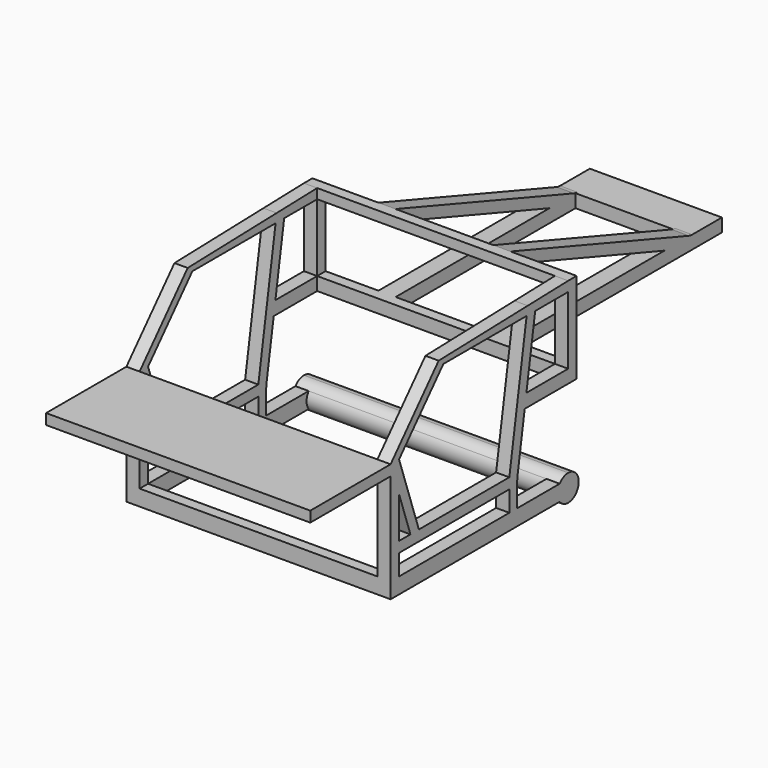
from build123d import *

# Parameters (mm, degrees)
F0_W     = 4
F0_H     = 6
F0_W_2   = 5.376602
F0_H_2   = 4
F0_W_3   = 3.587166
F0_H_3   = 7.83267
F0_H_4   = 5
F0_W_4   = 38
F1_DEPTH = 50
F2_DEPTH = 45
F3_DEPTH = 45
F4_DEPTH = 45
F5_DEPTH = 25
F6_DEPTH = 18.5
F7_W     = 14.907549
F7_H     = 5
F8_DEPTH = 37
F9_R     = 5


with BuildPart() as f1:
    # F0 (on Right) → F1 (new body, symmetric)
    with BuildSketch(Plane.YZ):
        Polygon((-49, -26), (-45, -26), (-45, -18.16733), (-45, -14.16733), (-45, 1.410587), (-49, 13), (-49, 9), align=None)
        with Locations((-47, -29)):
            Rectangle(F0_W, F0_H)
        Polygon((-26.269564, 38.284922), (-49, 13), (-45, 13), (-24.038542, 36.279295), align=None)
        Polygon((-24.038542, 36.279295), (15.345107, 36.279295), (15.861475, 39.464268), (-26.269564, 38.284922), align=None)
        Polygon((15.861475, 39.464268), (15.345107, 36.279295), (19.397336, 36.279295), (35, 36.279295), (35, 40), align=None)
        Polygon((-49, 13), (-45, 1.410587), (-45, 13), align=None)
        Polygon((-45, 1.410587), (-39.623398, -14.16733), (-35.623398, -14.16733), (-45, 13), align=None)
        Polygon((-39.623398, -18.16733), (7.166378, -18.16733), (7.166378, -14.16733), (-35.623398, -14.16733), (-39.623398, -14.16733), align=None)
        Polygon((7.166378, -18.16733), (10.753544, -18.16733), (11.114822, -14.807477), (7.166378, -14.16733), align=None)
        Polygon((7.166378, -14.16733), (11.114822, -14.807477), (14.437454, 5.686611), (15.248086, 10.686611), (19.397336, 36.279295), (15.345107, 36.279295), align=None)
        with Locations((-42.311699, -16.16733)):
            Rectangle(F0_W_2, F0_H_2)
        with Locations((8.959961, -22.083665)):
            Rectangle(F0_W_3, F0_H_3)
        Polygon((10.753544, -32), (10.753544, -26), (7.166378, -26), (-45, -26), (-45, -32), align=None)
        with BuildLine():
            ThreePointArc((35, -24), (32.763932, -24.527864), (31, -26))
            Line((31, -26), (35, -26))
            Line((35, -26), (35, -24))
        make_face()
        with BuildLine():
            Line((35, -26), (31, -26))
            ThreePointArc((31, -26), (30, -29), (31, -32))
            Line((31, -32), (35, -32))
            Line((35, -32), (35, -26))
        make_face()
        with BuildLine():
            Line((35, -32), (31, -32))
            ThreePointArc((31, -32), (35, -34), (39, -32))
            Line((39, -32), (35, -32))
        make_face()
        with Locations((37, -29)):
            Rectangle(F0_W, F0_H)
        with BuildLine():
            Line((35, -24), (35, -26))
            Line((35, -26), (39, -26))
            ThreePointArc((39, -26), (37.236068, -24.527864), (35, -24))
        make_face()
        with BuildLine():
            ThreePointArc((40, -29), (39.743416, -27.418861), (39, -26))
            Line((39, -26), (39, -32))
            ThreePointArc((39, -32), (39.743416, -30.581139), (40, -29))
        make_face()
        with BuildLine():
            Line((31, -26), (10.753544, -26))
            Line((10.753544, -26), (10.753544, -32))
            Line((10.753544, -32), (31, -32))
            ThreePointArc((31, -32), (30, -29), (31, -26))
        make_face()
        Polygon((14.437454, 5.686611), (35, 5.686611), (35, 10.686611), (15.248086, 10.686611), align=None)
        Polygon((35, 40), (35, 36.279295), (39, 35.769307), (39, 40), align=None)
        with Locations((37, 8.186611)):
            Rectangle(F0_W, F0_H_4)
        with Locations((-68, 11)):
            Rectangle(F0_W_4, F0_H_2)
        Polygon((35, 36.279295), (35, 10.686611), (39, 10.686611), (39, 35.769307), align=None)
    extrude(amount=F1_DEPTH, both=True)

    # F0 (on Right) → F2 (cut, symmetric)
    with BuildSketch(Plane.YZ):
        Polygon((35, 36.279295), (35, 10.686611), (39, 10.686611), (39, 35.769307), align=None)
    extrude(amount=F2_DEPTH, both=True, mode=Mode.SUBTRACT)

    # F0 (on Right) → F3 (cut, symmetric)
    with BuildSketch(Plane.YZ):
        Polygon((7.166378, -14.16733), (11.114822, -14.807477), (14.437454, 5.686611), (15.248086, 10.686611), (19.397336, 36.279295), (15.345107, 36.279295), align=None)
        Polygon((-24.038542, 36.279295), (15.345107, 36.279295), (15.861475, 39.464268), (-26.269564, 38.284922), align=None)
        Polygon((15.861475, 39.464268), (15.345107, 36.279295), (19.397336, 36.279295), (35, 36.279295), (35, 40), align=None)
        Polygon((-26.269564, 38.284922), (-49, 13), (-45, 13), (-24.038542, 36.279295), align=None)
        Polygon((-49, 13), (-45, 1.410587), (-45, 13), align=None)
        Polygon((-45, 1.410587), (-39.623398, -14.16733), (-35.623398, -14.16733), (-45, 13), align=None)
        Polygon((-39.623398, -18.16733), (7.166378, -18.16733), (7.166378, -14.16733), (-35.623398, -14.16733), (-39.623398, -14.16733), align=None)
        Polygon((7.166378, -18.16733), (10.753544, -18.16733), (11.114822, -14.807477), (7.166378, -14.16733), align=None)
        with Locations((-42.311699, -16.16733)):
            Rectangle(F0_W_2, F0_H_2)
        with Locations((8.959961, -22.083665)):
            Rectangle(F0_W_3, F0_H_3)
        Polygon((10.753544, -32), (10.753544, -26), (7.166378, -26), (-45, -26), (-45, -32), align=None)
        with BuildLine():
            Line((31, -26), (10.753544, -26))
            Line((10.753544, -26), (10.753544, -32))
            Line((10.753544, -32), (31, -32))
            ThreePointArc((31, -32), (30, -29), (31, -26))
        make_face()
        Polygon((14.437454, 5.686611), (35, 5.686611), (35, 10.686611), (15.248086, 10.686611), align=None)
    extrude(amount=F3_DEPTH, both=True, mode=Mode.SUBTRACT)

    # F0 (on Right) → F4 (cut, symmetric)
    with BuildSketch(Plane.YZ):
        Polygon((-49, -26), (-45, -26), (-45, -18.16733), (-45, -14.16733), (-45, 1.410587), (-49, 13), (-49, 9), align=None)
    extrude(amount=F4_DEPTH, both=True, mode=Mode.SUBTRACT)

    # F0 (on Right) → F5 (join, symmetric)
    with BuildSketch(Plane.YZ):
        Polygon((39, 10.686611), (39, 5.686611), (139, 5.686611), (139, 10.686611), (124.092451, 10.686611), (39, 40), (39, 35.769307), (111.811374, 10.686611), align=None)
    extrude(amount=F5_DEPTH, both=True)

    # F0 (on Right) → F6 (cut, symmetric)
    with BuildSketch(Plane.YZ):
        Polygon((39, 10.686611), (39, 5.686611), (139, 5.686611), (139, 10.686611), (124.092451, 10.686611), (39, 40), (39, 35.769307), (111.811374, 10.686611), align=None)
    extrude(amount=F6_DEPTH, both=True, mode=Mode.SUBTRACT)

    # F7 (on face) → F8 (join, through all)
    with BuildSketch(Plane.YZ.offset(-18.5)):
        with Locations((131.546225, 8.186611)):
            Rectangle(F7_W, F7_H)
    extrude(amount=F8_DEPTH)

    # F9
    f9_edges = [f1.edges().sort_by_distance(p)[0] for p in [
        (-21.75, 124.092451, 10.686611),
        (21.75, 124.092451, 10.686611),
    ]]
    fillet(f9_edges, radius=F9_R)


solid = f1.part
